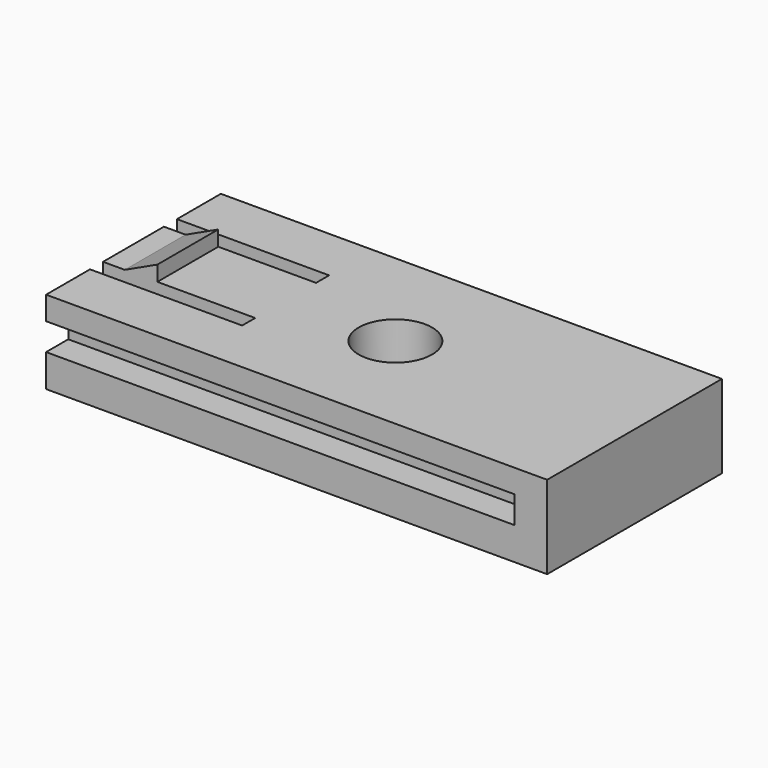
from build123d import *

# Parameters (mm, degrees)
F2_DEPTH        = 2.15
F3_W            = 3
F3_H            = 7
F4_DEPTH        = 1.4
F5_SIZE2        = 1.39999
F5_SIZE         = 2.99999
F6_W            = 3
F6_H            = 2.55
F7_DEPTH        = 2.5
F8_W            = 43.1
F8_H            = 2.55
F9_DEPTH        = 3
F11_D           = 4
F11_CBORE_D     = 6.75
F11_CBORE_DEPTH = 5.5


# Not quite as in the source:
# - a fillet or chamfer is up to 0.001 mm smaller than in the source, because OpenCascade refuses the exact size


with BuildPart() as f2:
    # F1 (on Top) → F2 (new body)
    with BuildSketch(Plane.XY):
        Polygon((-23.05, -5), (-23.05, -10.05), (23.05, -10.05), (23.05, 10.05), (-23.05, 10.05), (-23.05, 5), (-9.05, 5), (-9.05, 3.5), (-23.05, 3.5), (-23.05, -3.5), (-9.05, -3.5), (-9.05, -5), align=None)
    extrude(amount=F2_DEPTH)

    # F3 (on face) → F4 (join)
    with BuildSketch(Plane.XY.offset(2.15)):
        with Locations((-19.55, 0)):
            Rectangle(F3_W, F3_H)
    extrude(amount=F4_DEPTH)

    # F5 (size 3 and 1.4 in the source; OpenCascade refuses exactly that, so slightly less here)
    f5_edges = [f2.edges().sort_by_distance(p)[0] for p in [
        (-21.05, 0, 3.55),
    ]]
    f5_side = f2.faces().sort_by_distance((-19.55, 0, 3.55))[0]
    chamfer(f5_edges, length=F5_SIZE, length2=F5_SIZE2, reference=f5_side)

    # F6 (on face) → F7 (join)
    with BuildSketch(Plane(origin=(0, 0, 0), x_dir=(1, 0, 0), z_dir=(0, 0, -1))):
        Polygon((-23.05, -5), (-23.05, -7.5), (20.05, -7.5), (23.05, -7.5), (23.05, 7.5), (20.05, 7.5), (-23.05, 7.5), (-23.05, 5), (-9.05, 5), (-9.05, 3.5), (-9.05, -3.5), (-9.05, -5), align=None)
        with Locations((21.55, 8.775)):
            Rectangle(F6_W, F6_H)
        with Locations((21.55, -8.775)):
            Rectangle(F6_W, F6_H)
    extrude(amount=F7_DEPTH)

    # F8 (on face) → F9 (join)
    with BuildSketch(Plane(origin=(0, 0, -2.5), x_dir=(1, 0, 0), z_dir=(0, 0, -1))):
        Polygon((23.05, -10.05), (23.05, 10.05), (20.05, 10.05), (20.05, 7.5), (-23.05, 7.5), (-23.05, 5), (-9.05, 5), (-9.05, -5), (-23.05, -5), (-23.05, -7.5), (20.05, -7.5), (20.05, -10.05), align=None)
        with Locations((-1.5, -8.775)):
            Rectangle(F8_W, F8_H)
        with Locations((-1.5, 8.775)):
            Rectangle(F8_W, F8_H)
    extrude(amount=F9_DEPTH)

    # F11 (through all)
    with Locations(Plane.XY.offset(2.15)):
        with Locations((1.05, 0)):
            CounterBoreHole(F11_D / 2, F11_CBORE_D / 2, F11_CBORE_DEPTH)


solid = f2.part
